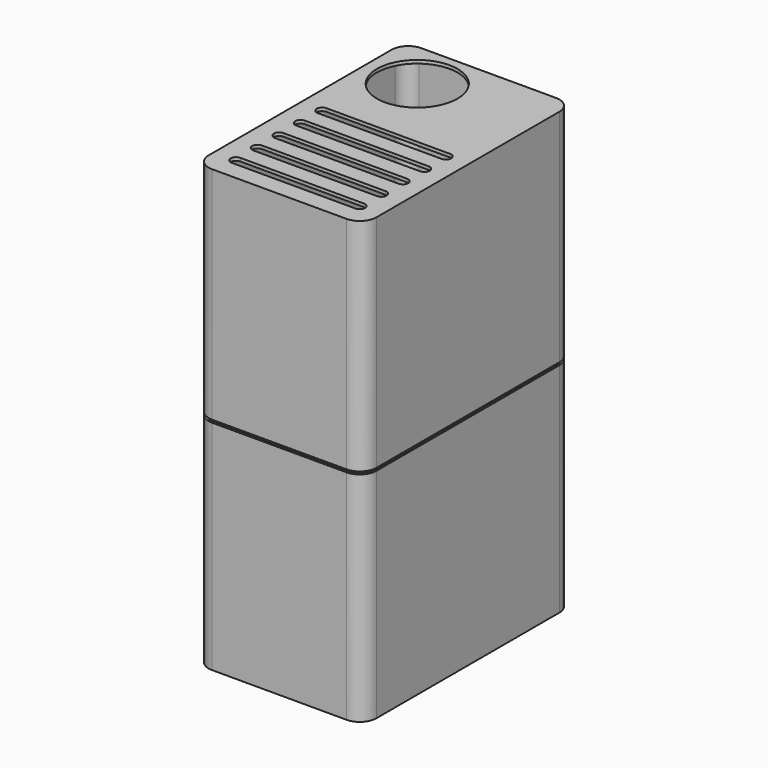
from build123d import *

# Parameters (mm, degrees)
F1_DEPTH  = 82
F2_DEPTH  = 1.2
F4_DEPTH  = 1
F7_DEPTH  = 1
F8_DEPTH  = 1
F9_R      = 15
F10_DEPTH = 1.2


# Not quite as in the source:
# - a feature names something its author has since deleted; it is built from what else it names


with BuildPart() as f1:
    # F0 (on Top) → F1 (new body)
    with BuildSketch(Plane.XY):
        with BuildLine():
            Line((31.2, -42.5), (31.2, 42.5))
            ThreePointArc((31.2, 42.5), (29.3840620434, 46.8840620434), (25, 48.7))
            Line((25, 48.7), (-25, 48.7))
            ThreePointArc((-25, 48.7), (-29.3840620434, 46.8840620434), (-31.2, 42.5))
            Line((-31.2, 42.5), (-31.2, -42.5))
            ThreePointArc((-31.2, -42.5), (-29.3840620434, -46.8840620434), (-25, -48.7))
            Line((-25, -48.7), (25, -48.7))
            ThreePointArc((25, -48.7), (29.3840620434, -46.8840620434), (31.2, -42.5))
        make_face()
        with BuildLine():
            Line((-25, 47.5), (25, 47.5))
            ThreePointArc((25, 47.5), (28.5355339059, 46.0355339059), (30, 42.5))
            Line((30, 42.5), (30, -42.5))
            ThreePointArc((30, -42.5), (28.5355339059, -46.0355339059), (25, -47.5))
            Line((25, -47.5), (-25, -47.5))
            ThreePointArc((-25, -47.5), (-28.5355339059, -46.0355339059), (-30, -42.5))
            Line((-30, -42.5), (-30, 42.5))
            ThreePointArc((-30, 42.5), (-28.5355339059, 46.0355339059), (-25, 47.5))
        make_face(mode=Mode.SUBTRACT)
    extrude(amount=F1_DEPTH)

    # F0 (on Top) → F2 (join)
    with BuildSketch(Plane.XY):
        with BuildLine():
            ThreePointArc((30, 42.5), (28.5355339059, 46.0355339059), (25, 47.5))
            Line((25, 47.5), (-25, 47.5))
            ThreePointArc((-25, 47.5), (-28.5355339059, 46.0355339059), (-30, 42.5))
            Line((-30, 42.5), (-30, -42.5))
            ThreePointArc((-30, -42.5), (-28.5355339059, -46.0355339059), (-25, -47.5))
            Line((-25, -47.5), (25, -47.5))
            ThreePointArc((25, -47.5), (28.5355339059, -46.0355339059), (30, -42.5))
            Line((30, -42.5), (30, 42.5))
        make_face()
    extrude(amount=F2_DEPTH)

    # F3 (on face) → F4 (cut)
    with BuildSketch(Plane.XY.offset(82)):
        with BuildLine():
            ThreePointArc((25, -48.7), (29.3840620434, -46.8840620434), (31.2, -42.5))
            Line((31.2, -42.5), (31.2, 42.5))
            ThreePointArc((31.2, 42.5), (29.3840620434, 46.8840620434), (25, 48.7))
            Line((25, 48.7), (-25, 48.7))
            ThreePointArc((-25, 48.7), (-29.3840620434, 46.8840620434), (-31.2, 42.5))
            Line((-31.2, 42.5), (-31.2, -42.5))
            ThreePointArc((-31.2, -42.5), (-29.3840620434, -46.8840620434), (-25, -48.7))
            Line((-25, -48.7), (25, -48.7))
        make_face()
        with BuildLine():
            ThreePointArc((-25, -48), (-28.8890872965, -46.3890872965), (-30.5, -42.5))
            Line((-30.5, -42.5), (-30.5, 42.5))
            ThreePointArc((-30.5, 42.5), (-28.8890872965, 46.3890872965), (-25, 48))
            Line((-25, 48), (25, 48))
            ThreePointArc((25, 48), (28.8890872965, 46.3890872965), (30.5, 42.5))
            Line((30.5, 42.5), (30.5, -42.5))
            ThreePointArc((30.5, -42.5), (28.8890872965, -46.3890872965), (25, -48))
            Line((25, -48), (-25, -48))
        make_face(mode=Mode.SUBTRACT)
    extrude(amount=-F4_DEPTH, mode=Mode.SUBTRACT)


with BuildPart() as f5_1:
    # F5: instance of F1
    add(f1.part.mirror(Plane.XY.offset(82)))

    # F6 (on face) → F7 (join)
    with BuildSketch(Plane(origin=(0, 0, 83), x_dir=(1, 0, 0), z_dir=(0, 0, -1))):
        with BuildLine():
            Line((31.2, -42.5), (31.2, 42.5))
            ThreePointArc((31.2, 42.5), (29.3840620434, 46.8840620434), (25, 48.7))
            Line((25, 48.7), (-25, 48.7))
            ThreePointArc((-25, 48.7), (-29.3840620434, 46.8840620434), (-31.2, 42.5))
            Line((-31.2, 42.5), (-31.2, -42.5))
            ThreePointArc((-31.2, -42.5), (-29.3840620434, -46.8840620434), (-25, -48.7))
            Line((-25, -48.7), (25, -48.7))
            ThreePointArc((25, -48.7), (29.3840620434, -46.8840620434), (31.2, -42.5))
        make_face()
        with BuildLine():
            ThreePointArc((25, 48.2), (29.0305086528, 46.5305086528), (30.7, 42.5))
            Line((30.7, 42.5), (30.7, -42.5))
            ThreePointArc((30.7, -42.5), (29.0305086528, -46.5305086528), (25, -48.2))
            Line((25, -48.2), (-25, -48.2))
            ThreePointArc((-25, -48.2), (-29.0305086528, -46.5305086528), (-30.7, -42.5))
            Line((-30.7, -42.5), (-30.7, 42.5))
            ThreePointArc((-30.7, 42.5), (-29.0305086528, 46.5305086528), (-25, 48.2))
            Line((-25, 48.2), (25, 48.2))
        make_face(mode=Mode.SUBTRACT)
    extrude(amount=F7_DEPTH)

    # F8 (cut): a face of the model
    f8_faces = [f5_1.faces().sort_by_distance(p)[0] for p in [
        (28.808660311, -46.308660311, 82),
    ]]
    extrude(f8_faces, amount=-F8_DEPTH, mode=Mode.SUBTRACT)

    # F9 (on face) → F10 (cut)
    with BuildSketch(Plane.XY.offset(164)):
        with Locations((-12.0217995225, 30.4631138757)):
            Circle(F9_R)
        with BuildLine():
            ThreePointArc((25, 0), (24.4142135624, 1.4142135624), (23, 2))
            Line((23, 2), (-23, 2))
            ThreePointArc((-23, 2), (-24.4142135624, 1.4142135624), (-25, 0))
            ThreePointArc((-25, 0), (-24.4142135624, -1.4142135624), (-23, -2))
            Line((-23, -2), (23, -2))
            ThreePointArc((23, -2), (24.4142135624, -1.4142135624), (25, 0))
        make_face()
        with BuildLine():
            ThreePointArc((-23, -8), (-24.4142135624, -8.5857864376), (-25, -10))
            ThreePointArc((-25, -10), (-24.4142135624, -11.4142135624), (-23, -12))
            Line((-23, -12), (23, -12))
            ThreePointArc((23, -12), (24.4142135624, -11.4142135624), (25, -10))
            ThreePointArc((25, -10), (24.4142135624, -8.5857864376), (23, -8))
            Line((23, -8), (-23, -8))
        make_face()
        with BuildLine():
            ThreePointArc((-23, -18), (-24.4142135624, -18.5857864376), (-25, -20))
            ThreePointArc((-25, -20), (-24.4142135624, -21.4142135624), (-23, -22))
            Line((-23, -22), (23, -22))
            ThreePointArc((23, -22), (24.4142135624, -21.4142135624), (25, -20))
            ThreePointArc((25, -20), (24.4142135624, -18.5857864376), (23, -18))
            Line((23, -18), (-23, -18))
        make_face()
        with BuildLine():
            ThreePointArc((-23, -28), (-24.4142135624, -28.5857864376), (-25, -30))
            ThreePointArc((-25, -30), (-24.4142135624, -31.4142135624), (-23, -32))
            Line((-23, -32), (23, -32))
            ThreePointArc((23, -32), (24.4142135624, -31.4142135624), (25, -30))
            ThreePointArc((25, -30), (24.4142135624, -28.5857864376), (23, -28))
            Line((23, -28), (-23, -28))
        make_face()
        with BuildLine():
            ThreePointArc((-23, -38), (-24.4142135624, -38.5857864376), (-25, -40))
            ThreePointArc((-25, -40), (-24.4142135624, -41.4142135624), (-23, -42))
            Line((-23, -42), (23, -42))
            ThreePointArc((23, -42), (24.4142135624, -41.4142135624), (25, -40))
            ThreePointArc((25, -40), (24.4142135624, -38.5857864376), (23, -38))
            Line((23, -38), (-23, -38))
        make_face()
    extrude(amount=-F10_DEPTH, mode=Mode.SUBTRACT)


solid = Compound([f1.part, f5_1.part])
